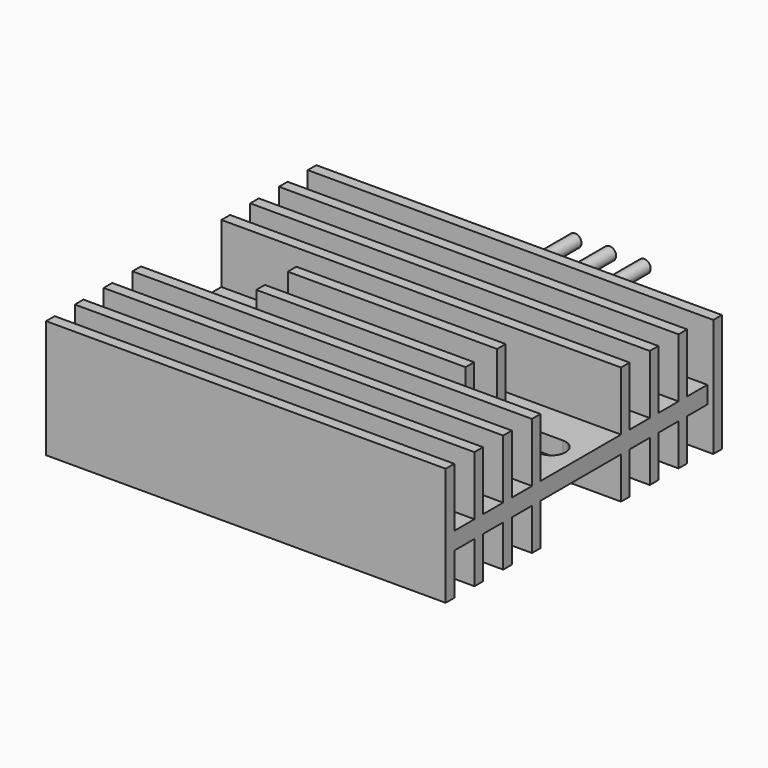
from build123d import *

# Parameters (mm, degrees)
F0_W     = 94.5642
F0_H     = 79.9338
F1_DEPTH = 4.1148
F2_W     = 22.5171
F2_H     = 2.54
F2_W_2   = 49.53
F2_W_3   = 1.4234517733
F3_DEPTH = 13.97
F4_W     = 32.766
F4_H     = 15.24
F5_DEPTH = 2.286
F7_W     = 49.53
F7_H     = 5.969
F7_H_2   = 2.54
F7_H_3   = 6.7818
F8_DEPTH = 9.779
F6_R     = 1.524
F9_DEPTH = 25.4


with BuildPart() as f1:
    # F0 (on Top) → F1 (new body)
    with BuildSketch(Plane.XY):
        Rectangle(F0_W, F0_H)
        with BuildLine():
            Line((-40.3606, 3.3655), (-33.5026, 3.3655))
            ThreePointArc((-33.5026, 3.3655), (-30.1371, 0), (-33.5026, -3.3655))
            Line((-33.5026, -3.3655), (-40.3606, -3.3655))
            ThreePointArc((-40.3606, -3.3655), (-43.7261, 0), (-40.3606, 3.3655))
        make_face(mode=Mode.SUBTRACT)
        with BuildLine():
            Line((33.5026, 3.3655), (40.3606, 3.3655))
            ThreePointArc((40.3606, 3.3655), (43.7134059906, -0.0063380302), (40.3479, -3.3655))
            Line((40.3479, -3.3655), (33.4899, -3.3655))
            ThreePointArc((33.4899, -3.3655), (30.1243940094, 0.0063619924), (33.5026, 3.3655))
        make_face(mode=Mode.SUBTRACT)
    extrude(amount=F1_DEPTH)

    # F2 (on face) → F3 (join, symmetric)
    with BuildSketch(Plane.XY.offset(4.1148)):
        with Locations((36.02355, -38.6969)):
            Rectangle(F2_W, F2_H)
        with Locations((-36.02355, 38.6969)):
            Rectangle(F2_W, F2_H)
        with Locations((-36.02355, -38.6969)):
            Rectangle(F2_W, F2_H)
        with Locations((0, 38.6969)):
            Rectangle(F2_W_2, F2_H)
        with Locations((36.02355, 30.1879)):
            Rectangle(F2_W, F2_H)
        with Locations((36.02355, 21.6789)):
            Rectangle(F2_W, F2_H)
        with Locations((36.02355, 13.1699)):
            Rectangle(F2_W, F2_H)
        with Locations((36.02355, -13.1699)):
            Rectangle(F2_W, F2_H)
        with Locations((36.02355, -21.6789)):
            Rectangle(F2_W, F2_H)
        with Locations((36.02355, -30.1879)):
            Rectangle(F2_W, F2_H)
        with Locations((0, -38.6969)):
            Rectangle(F2_W_2, F2_H)
        with Locations((-36.02355, 30.1879)):
            Rectangle(F2_W, F2_H)
        with Locations((-36.02355, 21.6789)):
            Rectangle(F2_W, F2_H)
        with Locations((-36.02355, 13.1699)):
            Rectangle(F2_W, F2_H)
        with Locations((-36.02355, -13.1699)):
            Rectangle(F2_W, F2_H)
        with Locations((-36.02355, -21.6789)):
            Rectangle(F2_W, F2_H)
        with Locations((-36.02355, -30.1879)):
            Rectangle(F2_W, F2_H)
        with Locations((0, 30.1879)):
            Rectangle(F2_W_2, F2_H)
        with Locations((0, 21.6789)):
            Rectangle(F2_W_2, F2_H)
        with Locations((0, 13.1699)):
            Rectangle(F2_W_2, F2_H)
        with Locations((0, -13.1699)):
            Rectangle(F2_W_2, F2_H)
        with Locations((0, -21.6789)):
            Rectangle(F2_W_2, F2_H)
        with Locations((0, -30.1879)):
            Rectangle(F2_W_2, F2_H)
        with Locations((0, 4.6609)):
            Rectangle(F2_W_2, F2_H)
        with Locations((0, -4.6609)):
            Rectangle(F2_W_2, F2_H)
        with Locations((47.9938258867, 38.6969)):
            Rectangle(F2_W_3, F2_H)
        with Locations((36.02355, 38.6969)):
            Rectangle(F2_W, F2_H)
    extrude(amount=F3_DEPTH, both=True)

    # F4 (on face) → F5 (join)
    with BuildSketch(Plane(origin=(0, 39.9669, 0), x_dir=(-1, 0, 0), z_dir=(0, 1, 0))):
        Rectangle(F4_W, F4_H)
    extrude(amount=F5_DEPTH)

    # F7 (on face) → F8 (join)
    with BuildSketch(Plane(origin=(0, 0, 0), x_dir=(1, 0, 0), z_dir=(0, 0, -1))):
        with Locations((0, 8.9154)):
            Rectangle(F7_W, F7_H)
        with Locations((0, 4.6609)):
            Rectangle(F7_W, F7_H_2)
        Rectangle(F7_W, F7_H_3)
        with Locations((0, -4.6609)):
            Rectangle(F7_W, F7_H_2)
        with Locations((0, -8.9154)):
            Rectangle(F7_W, F7_H)
    extrude(amount=F8_DEPTH)

    # F6 (on face) → F9 (join)
    with BuildSketch(Plane(origin=(0, 42.2529, 0), x_dir=(-1, 0, 0), z_dir=(0, 1, 0))):
        with Locations((-8.1915, 3.81)):
            Circle(F6_R)
        with Locations((8.1915, 3.81)):
            Circle(F6_R)
        with Locations((4.09575, 0)):
            Circle(F6_R)
        with Locations((-4.09575, 0)):
            Circle(F6_R)
        with Locations((8.1915, -3.7334442604)):
            Circle(F6_R)
        with Locations((-8.1915, -3.81)):
            Circle(F6_R)
        with Locations((0, 3.81)):
            Circle(F6_R)
        with Locations((0, -3.81)):
            Circle(F6_R)
    extrude(amount=F9_DEPTH)


solid = f1.part
